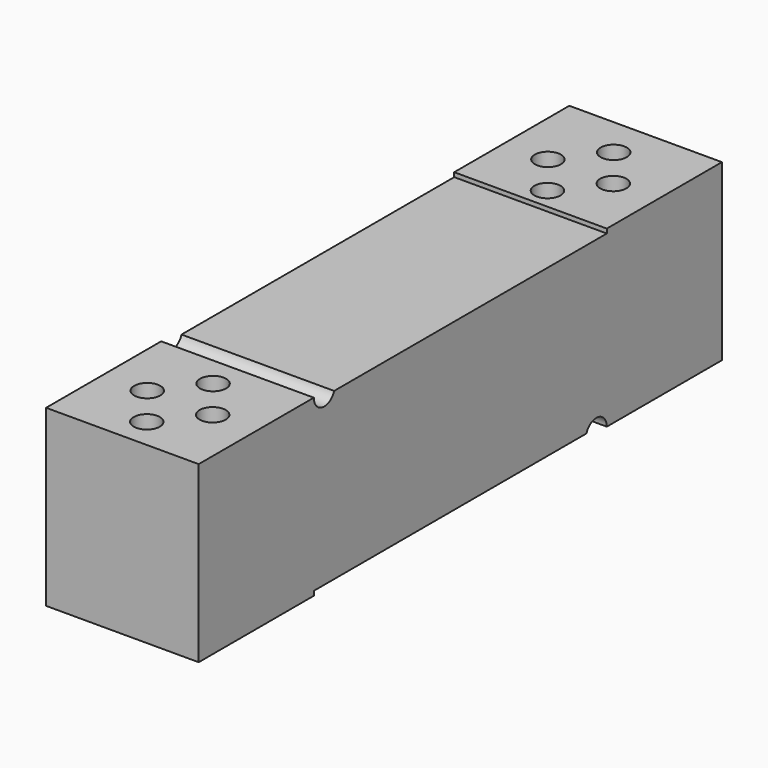
from build123d import *

# Parameters (mm, degrees)
F0_W     = 35
F0_H     = 150
F1_DEPTH = 20
F3_D     = 6
F5_DEPTH = 25


# Not quite as in the source:
# - a pattern or mirror of a feature is missing from the dataset's text; its kind, count and spacing are read off the source's solid


with BuildPart() as f1:
    # F0 (on Top) → F1 (new body, symmetric)
    with BuildSketch(Plane.XY):
        with Locations((0, 1.0728642344)):
            Rectangle(F0_W, F0_H)
    extrude(amount=F1_DEPTH, both=True)

    # F3 (through all)
    with Locations(Plane.XY.offset(20)):
        with Locations((0, -66.9271357656), (-7.5, -57.4271357656), (0, -47.9271357656), (7.5, -57.4271357656)):
            f3 = Hole(F3_D / 2)

    # F3_copies: F3 across plane
    add(f3.mirror(Plane.ZX), mode=Mode.SUBTRACT)

    # F4 (on Right) → F5 (cut, symmetric)
    with BuildSketch(Plane.YZ):
        with BuildLine():
            Line((43.0728642344, 20), (-37.8160246544, 22.9979416807))
            ThreePointArc((-37.8160246544, 22.9979416807), (-40.4082858377, 18.3136150145), (-35.0987086408, 19))
            Line((-35.0987086408, 19), (43.0728642344, 19))
            Line((43.0728642344, 19), (43.0728642344, 20))
        make_face()
        with BuildLine():
            Line((-40.9271357656, -20), (39.9617531233, -22.9979416807))
            ThreePointArc((39.9617531233, -22.9979416807), (42.5540143066, -18.3136150145), (37.2444371097, -19))
            Line((37.2444371097, -19), (-40.9271357656, -19))
            Line((-40.9271357656, -19), (-40.9271357656, -20))
        make_face()
    extrude(amount=F5_DEPTH, both=True, mode=Mode.SUBTRACT)


solid = f1.part
